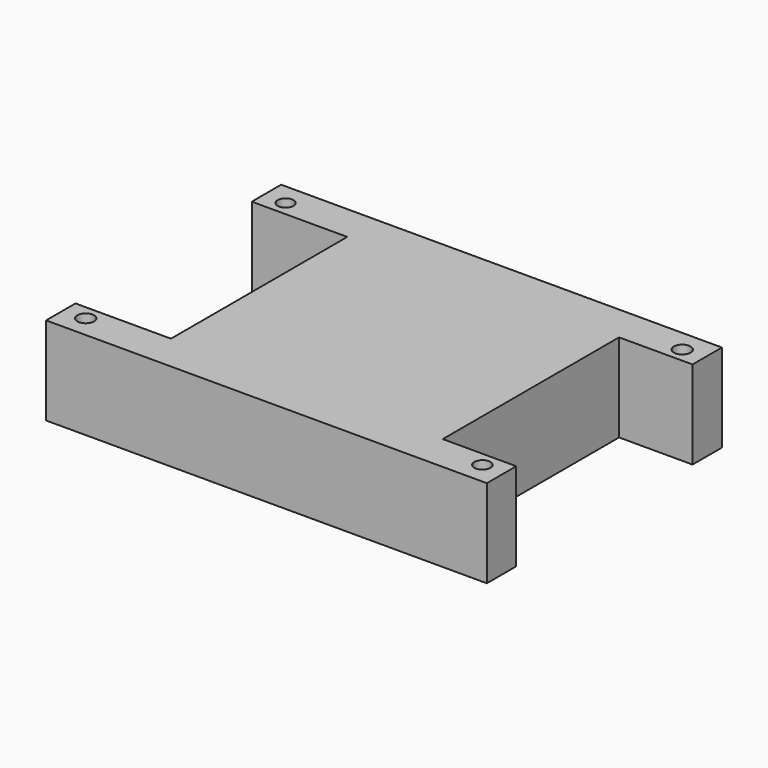
from build123d import *

# Parameters (mm, degrees)
F0_R        = 1.3671138527
F0_R_2      = 1.4471777078
F0_W        = 46.99
F0_H        = 38.1
F0_R_3      = 1.4536013708
F0_R_4      = 1.3946138209
F1_DEPTH    = 15.24
F2_T        = 2.54
F2_T3_DEPTH = 20.32


# Not quite as in the source:
# - a shell that OpenCascade refuses in one call is made with other operations: the cavity is built on its own and cut out


with BuildPart() as f1:
    # F0 (on Top) → F1 (new body)
    with BuildSketch(Plane.XY):
        Polygon((0, 46.99), (0, 44.45), (16.51, 44.45), (63.5, 44.45), (76.2, 44.45), (76.2, 46.99), (76.2, 50.8), (72.39, 50.8), (3.81, 50.8), (0, 50.8), align=None)
        with Locations((3.81, 46.99)):
            Circle(F0_R, mode=Mode.SUBTRACT)
        with Locations((72.39, 46.99)):
            Circle(F0_R_2, mode=Mode.SUBTRACT)
        with Locations((40.005, 25.4)):
            Rectangle(F0_W, F0_H)
        Polygon((0, 3.175), (0, 0), (3.81, 0), (72.39, 0), (76.2, 0), (76.2, 3.81), (76.2, 6.35), (63.5, 6.35), (16.51, 6.35), (0, 6.35), (0, 3.81), align=None)
        with Locations((3.81, 3.81)):
            Circle(F0_R_3, mode=Mode.SUBTRACT)
        with Locations((72.39, 3.81)):
            Circle(F0_R_4, mode=Mode.SUBTRACT)
    extrude(amount=F1_DEPTH)

    # F2: shell of thickness 2.54, made by hand


with BuildPart() as f2_core1:
    # F2_t2: copy of F1
    add(f1.part)

    # the walls: a layer under each face that stays
    f2_faces = [f2_core1.faces().sort_by_distance(p)[0] for p in [
        (8.255, 44.45, 7.62),
        (16.51, 25.4, 7.62),
        (8.255, 6.35, 7.62),
        (0, 3.175, 7.62),
        (38.1, 0, 7.62),
        (76.2, 3.175, 7.62),
        (69.85, 6.35, 7.62),
        (63.5, 25.4, 7.62),
        (69.85, 44.45, 7.62),
        (76.2, 47.625, 7.62),
        (38.1, 50.8, 7.62),
        (0, 47.625, 7.62),
        (2.4428861473, 46.99, 7.62),
        (70.9428222922, 46.99, 7.62),
        (70.9953861791, 3.81, 7.62),
        (2.3563986292, 3.81, 7.62),
        (38.1, 25.4, 15.24),
    ]]
    thicken(f2_faces, amount=-F2_T, mode=Mode.SUBTRACT)

    # F2_s4 → F2_t3 (cut)
    with BuildSketch(Plane.XY.offset(-2.54)):
        Polygon((16.4846, 44.4246), (16.51, 46.99), (19.05, 46.99), (19.05, 44.45), align=None)
        Polygon((16.4846, 6.3754), (19.05, 6.35), (19.05, 3.81), (16.51, 3.81), align=None)
        Polygon((63.5254, 6.3754), (63.5, 3.81), (60.96, 3.81), (60.96, 6.35), align=None)
        Polygon((63.5254, 44.4246), (60.96, 44.45), (60.96, 46.99), (63.5, 46.99), align=None)
    extrude(amount=F2_T3_DEPTH, mode=Mode.SUBTRACT)


with BuildPart() as f1_1:
    add(f1.part)

    # what is left inside the walls is the cavity
    f2_cavity = [f2_core1.part.solids().sort_by_distance(p)[0] for p in [
        (38.085466, 17.78, 0.0254),
    ]]
    add(f2_cavity, mode=Mode.SUBTRACT)


solid = f1_1.part
